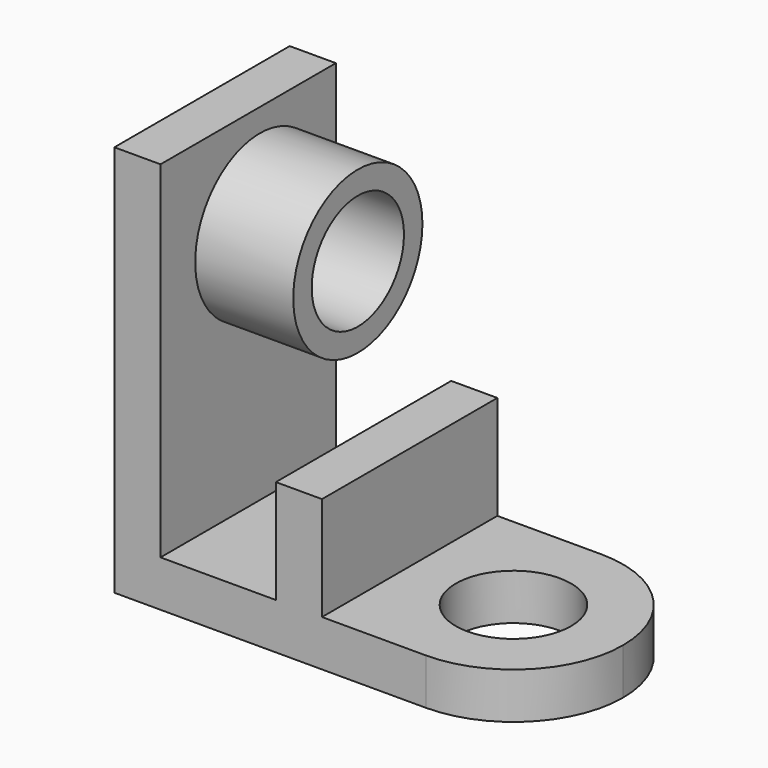
from build123d import *

# Parameters (mm, degrees)
F1_DEPTH = 19
F2_R     = 14
F2_R_2   = 10
F3_DEPTH = 17
F4_R     = 18.99999
F5_R     = 10
F6_DEPTH = 8.001
F7_W     = 8
F7_H     = 18
F8_DEPTH = 38


# Not quite as in the source:
# - a fillet or chamfer is up to 0.001 mm smaller than in the source, because OpenCascade refuses the exact size


with BuildPart() as f1:
    # F0 (on Front) → F1 (new body, symmetric)
    with BuildSketch(Plane.XZ):
        Polygon((0, 68), (0, 0), (73, 0), (73, 8), (8, 8), (8, 68), align=None)
    extrude(amount=F1_DEPTH, both=True)

    # F2 (on face) → F3 (join)
    with BuildSketch(Plane.YZ.offset(8)):
        with Locations((2.5166787673, 50)):
            Circle(F2_R)
        with Locations((2.5166787673, 50)):
            Circle(F2_R_2, mode=Mode.SUBTRACT)
    extrude(amount=F3_DEPTH)

    # F4 (radius 19 in the source; OpenCascade refuses exactly that, so slightly less here)
    f4_edges = [f1.edges().sort_by_distance(p)[0] for p in [
        (73, -19, 4),
        (73, 19, 4),
    ]]
    fillet(f4_edges, radius=F4_R)

    # F5 (on face) → F6 (cut, through all)
    with BuildSketch(Plane.XY.offset(8)):
        with Locations((54, 0)):
            Circle(F5_R)
    extrude(amount=-F6_DEPTH, mode=Mode.SUBTRACT)

    # F7 (on face) → F8 (join, through all)
    with BuildSketch(Plane.XZ.offset(19)):
        with Locations((32, 17)):
            Rectangle(F7_W, F7_H)
    extrude(amount=-F8_DEPTH)


solid = f1.part
